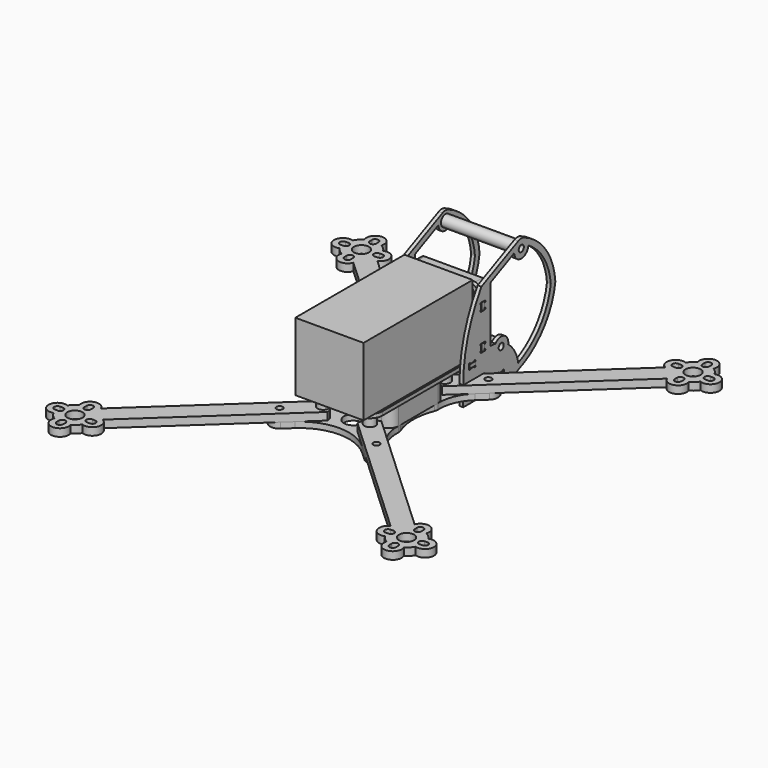
from build123d import *

# Parameters (mm, degrees)
F1_W      = 72
F1_H      = 36
F2_DEPTH  = 18
F4_R      = 1.7
F5_DEPTH  = 2
F7_R      = 1.7
F8_DEPTH  = 5
F13_R     = 1.7
F13_R_2   = 4
F14_DEPTH = 4
F16_R     = 1.7
F17_DEPTH = 10
F18_R     = 1.7
F18_R_2   = 5
F19_DEPTH = 3
F20_R     = 1.7
F21_DEPTH = 2
F24_R     = 1.7
F25_DEPTH = 2
F26_R     = 3
F26_R_2   = 1.7
F27_DEPTH = 6
F28_R     = 3
F28_R_2   = 1.7
F29_DEPTH = 38


# Not quite as in the source:
# - a feature names something its author has since deleted; it is built from what else it names


with BuildPart() as f2:
    # F1 (on Right) → F2 (new body, symmetric)
    with BuildSketch(Plane.YZ):
        with Locations((0, 23)):
            Rectangle(F1_W, F1_H)
    extrude(amount=F2_DEPTH, both=True)


with BuildPart() as f5:
    # F4 (on offset) → F5 (new body)
    with BuildSketch(Plane(origin=(0, 38, 0), x_dir=(-1, 0, 0), z_dir=(0, 1, 0))):
        with BuildLine():
            ThreePointArc((-15.25, 38), (-17.9016504294, 36.9016504294), (-19, 34.25))
            Line((-19, 34.25), (-19, 31.55))
            ThreePointArc((-19, 31.55), (-18.5, 31.05), (-19, 30.55))
            Line((-19, 30.55), (-21, 30.55))
            Line((-21, 30.55), (-21, 26.55))
            Line((-21, 26.55), (-19, 26.55))
            ThreePointArc((-19, 26.55), (-18.5, 26.05), (-19, 25.55))
            Line((-19, 25.55), (-19, 12.45))
            ThreePointArc((-19, 12.45), (-18.5, 11.95), (-19, 11.45))
            Line((-19, 11.45), (-21, 11.45))
            Line((-21, 11.45), (-21, 7.45))
            Line((-21, 7.45), (-19, 7.45))
            ThreePointArc((-19, 7.45), (-18.5, 6.95), (-19, 6.45))
            Line((-19, 6.45), (-19, 3.75))
            ThreePointArc((-19, 3.75), (-17.9016504294, 1.0983495706), (-15.25, 0))
            Line((-15.25, 0), (15.25, 0))
            ThreePointArc((15.25, 0), (17.9016504294, 1.0983495706), (19, 3.75))
            Line((19, 3.75), (19, 6.45))
            ThreePointArc((19, 6.45), (18.5, 6.95), (19, 7.45))
            Line((19, 7.45), (21, 7.45))
            Line((21, 7.45), (21, 11.45))
            Line((21, 11.45), (19, 11.45))
            ThreePointArc((19, 11.45), (18.5, 11.95), (19, 12.45))
            Line((19, 12.45), (19, 25.55))
            ThreePointArc((19, 25.55), (18.5, 26.05), (19, 26.55))
            Line((19, 26.55), (21, 26.55))
            Line((21, 26.55), (21, 30.55))
            Line((21, 30.55), (19, 30.55))
            ThreePointArc((19, 30.55), (18.5, 31.05), (19, 31.55))
            Line((19, 31.55), (19, 34.25))
            ThreePointArc((19, 34.25), (17.9016504294, 36.9016504294), (15.25, 38))
            Line((15.25, 38), (-15.25, 38))
        make_face()
        with Locations((-15.25, 3.75)):
            Circle(F4_R, mode=Mode.SUBTRACT)
        with Locations((15.25, 3.75)):
            Circle(F4_R, mode=Mode.SUBTRACT)
        with Locations((-15.25, 34.25)):
            Circle(F4_R, mode=Mode.SUBTRACT)
        with BuildLine():
            ThreePointArc((11.55, 34.25), (12.6337049096, 31.6337049096), (15.25, 30.55))
            Line((15.25, 30.55), (15.25, 7.45))
            ThreePointArc((15.25, 7.45), (12.6337049096, 6.3662950904), (11.55, 3.75))
            Line((11.55, 3.75), (-11.55, 3.75))
            ThreePointArc((-11.55, 3.75), (-12.6337049096, 6.3662950904), (-15.25, 7.45))
            Line((-15.25, 7.45), (-15.25, 30.55))
            ThreePointArc((-15.25, 30.55), (-12.6337049096, 31.6337049096), (-11.55, 34.25))
            Line((-11.55, 34.25), (11.55, 34.25))
        make_face(mode=Mode.SUBTRACT)
        with Locations((15.25, 34.25)):
            Circle(F4_R, mode=Mode.SUBTRACT)
    extrude(amount=F5_DEPTH)


with BuildPart() as f8:
    # F7 (on offset) → F8 (new body)
    with BuildSketch(Plane(origin=(0, 41, 0), x_dir=(-1, 0, 0), z_dir=(0, 1, 0))):
        with BuildLine():
            Line((15.25, 37), (-15.25, 37))
            ThreePointArc((-15.25, 37), (-17.1945436483, 36.1945436483), (-18, 34.25))
            Line((-18, 34.25), (-18, 3.75))
            ThreePointArc((-18, 3.75), (-17.1945436483, 1.8054563517), (-15.25, 1))
            Line((-15.25, 1), (15.25, 1))
            ThreePointArc((15.25, 1), (17.1945436483, 1.8054563517), (18, 3.75))
            Line((18, 3.75), (18, 34.25))
            ThreePointArc((18, 34.25), (17.1945436483, 36.1945436483), (15.25, 37))
        make_face()
        with Locations((-15.25, 3.75)):
            Circle(F7_R, mode=Mode.SUBTRACT)
        with Locations((15.25, 3.75)):
            Circle(F7_R, mode=Mode.SUBTRACT)
        with Locations((-15.25, 34.25)):
            Circle(F7_R, mode=Mode.SUBTRACT)
        with Locations((15.25, 34.25)):
            Circle(F7_R, mode=Mode.SUBTRACT)
    extrude(amount=F8_DEPTH)


with BuildPart() as f14:
    # F13 (on offset) → F14 (new body)
    with BuildSketch(Plane.XY.offset(-7)):
        with BuildLine():
            ThreePointArc((-13.5098647602, 23.45698286), (-13.5985378068, 25.8595100899), (-11.1960105769, 25.9481831366))
            Line((-11.1960105769, 25.9481831366), (-9.9504104386, 24.7912560449))
            ThreePointArc((-9.9504104386, 24.7912560449), (-8.9755957865, 24.5682394669), (-8.2950504384, 25.3009454306))
            Line((-8.2950504384, 25.3009454306), (-7.8315191856, 27.3270596371))
            Line((-7.8315191856, 27.3270596371), (-75.9697620511, 90.6146081253))
            ThreePointArc((-75.9697620511, 90.6146081253), (-77.7162022684, 90.1593612116), (-79.5054433115, 90.3958346237))
            ThreePointArc((-79.5054433115, 90.3958346237), (-80.9155407992, 88.3842819624), (-82.8176737402, 86.8297372354))
            ThreePointArc((-82.8176737402, 86.8297372354), (-82.4499479109, 85.0627961216), (-82.7752155315, 83.2875484882))
            Line((-82.7752155315, 83.2875484882), (-14.6369726661, 20))
            Line((-14.6369726661, 20), (-12.6505406659, 20.6116272629))
            ThreePointArc((-12.6505406659, 20.6116272629), (-11.9699953178, 21.3443332266), (-12.2642646219, 22.3000557683))
            Line((-12.2642646219, 22.3000557683), (-13.5098647602, 23.45698286))
        make_face()
        with Locations((-25.5416450153, 36.952399263)):
            Circle(F13_R, mode=Mode.SUBTRACT)
        with BuildLine():
            ThreePointArc((-79.5054433115, 90.3958346237), (-77.7162022684, 90.1593612116), (-75.9697620511, 90.6146081253))
            ThreePointArc((-75.9697620511, 90.6146081253), (-73.721275903, 96.7809760114), (-79.8297372354, 99.1823262598))
            ThreePointArc((-79.8297372354, 99.1823262598), (-81.3842819624, 101.0844592008), (-83.3958346237, 102.4945566885))
            ThreePointArc((-83.3958346237, 102.4945566885), (-88.0237403757, 108.6903381221), (-92.1823262598, 102.1702627646))
            ThreePointArc((-92.1823262598, 102.1702627646), (-94.0844592008, 100.6157180376), (-95.4945566885, 98.6041653763))
            ThreePointArc((-95.4945566885, 98.6041653763), (-101.6903381221, 93.9762596243), (-95.1702627646, 89.8176737402))
            ThreePointArc((-95.1702627646, 89.8176737402), (-93.6157180376, 87.9155407992), (-91.6041653763, 86.5054433115))
            ThreePointArc((-91.6041653763, 86.5054433115), (-88.7590568602, 80.5906195275), (-82.7752155315, 83.2875484882))
            ThreePointArc((-82.7752155315, 83.2875484882), (-82.4499479109, 85.0627961216), (-82.8176737402, 86.8297372354))
            ThreePointArc((-82.8176737402, 86.8297372354), (-80.9155407992, 88.3842819624), (-79.5054433115, 90.3958346237))
        make_face()
        with BuildLine():
            ThreePointArc((-96.930834755, 92.4507670157), (-98.6923793639, 94.0869089994), (-97.0562373802, 95.8484536083))
            Line((-97.0562373802, 95.8484536083), (-95.5572580011, 95.9037782959))
            ThreePointArc((-95.5572580011, 95.9037782959), (-93.7957133922, 94.2676363122), (-95.4318553759, 92.5060917033))
            Line((-95.4318553759, 92.5060917033), (-96.930834755, 92.4507670157))
        make_face(mode=Mode.SUBTRACT)
        with BuildLine():
            ThreePointArc((-85.4507670157, 85.069165245), (-87.0869089994, 83.3076206361), (-88.8484536083, 84.9437626198))
            Line((-88.8484536083, 84.9437626198), (-88.9037782959, 86.4427419989))
            ThreePointArc((-88.9037782959, 86.4427419989), (-87.2676363122, 88.2042866078), (-85.5060917033, 86.5681446241))
            Line((-85.5060917033, 86.5681446241), (-85.4507670157, 85.069165245))
        make_face(mode=Mode.SUBTRACT)
        with Locations((-87.5, 94.5)):
            Circle(F13_R_2, mode=Mode.SUBTRACT)
        with BuildLine():
            ThreePointArc((-78.069165245, 96.5492329843), (-76.3076206361, 94.9130910006), (-77.9437626198, 93.1515463917))
            Line((-77.9437626198, 93.1515463917), (-79.4427419989, 93.0962217041))
            ThreePointArc((-79.4427419989, 93.0962217041), (-81.2042866078, 94.7323636878), (-79.5681446241, 96.4939082967))
            Line((-79.5681446241, 96.4939082967), (-78.069165245, 96.5492329843))
        make_face(mode=Mode.SUBTRACT)
        with BuildLine():
            Line((-89.4939082967, 102.4318553759), (-89.5492329843, 103.930834755))
            ThreePointArc((-89.5492329843, 103.930834755), (-87.9130910006, 105.6923793639), (-86.1515463917, 104.0562373802))
            Line((-86.1515463917, 104.0562373802), (-86.0962217041, 102.5572580011))
            ThreePointArc((-86.0962217041, 102.5572580011), (-87.7323636878, 100.7957133922), (-89.4939082967, 102.4318553759))
        make_face(mode=Mode.SUBTRACT)
    extrude(amount=F14_DEPTH)


with BuildPart() as f14b:
    # F13 (on offset) → F14, piece 2 (new body)
    with BuildSketch(Plane.XY.offset(-7)):
        with BuildLine():
            Line((75.9697620511, 90.6146081253), (7.8315191856, 27.3270596371))
            Line((7.8315191856, 27.3270596371), (8.2950504384, 25.3009454306))
            ThreePointArc((8.2950504384, 25.3009454306), (8.9755957865, 24.5682394669), (9.9504104386, 24.7912560449))
            Line((9.9504104386, 24.7912560449), (11.1960105769, 25.9481831366))
            ThreePointArc((11.1960105769, 25.9481831366), (13.5985378068, 25.8595100899), (13.5098647602, 23.45698286))
            Line((13.5098647602, 23.45698286), (12.2642646219, 22.3000557683))
            ThreePointArc((12.2642646219, 22.3000557683), (11.9699953178, 21.3443332266), (12.6505406659, 20.6116272629))
            Line((12.6505406659, 20.6116272629), (14.6369726661, 20))
            Line((14.6369726661, 20), (82.7752155315, 83.2875484882))
            ThreePointArc((82.7752155315, 83.2875484882), (82.4499479109, 85.0627961216), (82.8176737402, 86.8297372354))
            ThreePointArc((82.8176737402, 86.8297372354), (80.9155407992, 88.3842819624), (79.5054433115, 90.3958346237))
            ThreePointArc((79.5054433115, 90.3958346237), (77.7162022684, 90.1593612116), (75.9697620511, 90.6146081253))
        make_face()
        with Locations((25.5416450153, 36.952399263)):
            Circle(F13_R, mode=Mode.SUBTRACT)
        with BuildLine():
            ThreePointArc((79.8297372354, 99.1823262598), (73.721275903, 96.7809760114), (75.9697620511, 90.6146081253))
            ThreePointArc((75.9697620511, 90.6146081253), (77.7162022684, 90.1593612116), (79.5054433115, 90.3958346237))
            ThreePointArc((79.5054433115, 90.3958346237), (80.9155407992, 88.3842819624), (82.8176737402, 86.8297372354))
            ThreePointArc((82.8176737402, 86.8297372354), (82.4499479109, 85.0627961216), (82.7752155315, 83.2875484882))
            ThreePointArc((82.7752155315, 83.2875484882), (88.7590568602, 80.5906195275), (91.6041653763, 86.5054433115))
            ThreePointArc((91.6041653763, 86.5054433115), (93.6157180376, 87.9155407992), (95.1702627646, 89.8176737402))
            ThreePointArc((95.1702627646, 89.8176737402), (101.6903381221, 93.9762596243), (95.4945566885, 98.6041653763))
            ThreePointArc((95.4945566885, 98.6041653763), (94.0844592008, 100.6157180376), (92.1823262598, 102.1702627646))
            ThreePointArc((92.1823262598, 102.1702627646), (88.0237403757, 108.6903381221), (83.3958346237, 102.4945566885))
            ThreePointArc((83.3958346237, 102.4945566885), (81.3842819624, 101.0844592008), (79.8297372354, 99.1823262598))
        make_face()
        with BuildLine():
            Line((88.9037782959, 86.4427419989), (88.8484536083, 84.9437626198))
            ThreePointArc((88.8484536083, 84.9437626198), (87.0869089994, 83.3076206361), (85.4507670157, 85.069165245))
            Line((85.4507670157, 85.069165245), (85.5060917033, 86.5681446241))
            ThreePointArc((85.5060917033, 86.5681446241), (87.2676363122, 88.2042866078), (88.9037782959, 86.4427419989))
        make_face(mode=Mode.SUBTRACT)
        with BuildLine():
            Line((78.069165245, 96.5492329843), (79.5681446241, 96.4939082967))
            ThreePointArc((79.5681446241, 96.4939082967), (81.2042866078, 94.7323636878), (79.4427419989, 93.0962217041))
            Line((79.4427419989, 93.0962217041), (77.9437626198, 93.1515463917))
            ThreePointArc((77.9437626198, 93.1515463917), (76.3076206361, 94.9130910006), (78.069165245, 96.5492329843))
        make_face(mode=Mode.SUBTRACT)
        with Locations((87.5, 94.5)):
            Circle(F13_R_2, mode=Mode.SUBTRACT)
        with BuildLine():
            Line((95.5572580011, 95.9037782959), (97.0562373802, 95.8484536083))
            ThreePointArc((97.0562373802, 95.8484536083), (98.6923793639, 94.0869089994), (96.930834755, 92.4507670157))
            Line((96.930834755, 92.4507670157), (95.4318553759, 92.5060917033))
            ThreePointArc((95.4318553759, 92.5060917033), (93.7957133922, 94.2676363122), (95.5572580011, 95.9037782959))
        make_face(mode=Mode.SUBTRACT)
        with BuildLine():
            Line((86.0962217041, 102.5572580011), (86.1515463917, 104.0562373802))
            ThreePointArc((86.1515463917, 104.0562373802), (87.9130910006, 105.6923793639), (89.5492329843, 103.930834755))
            Line((89.5492329843, 103.930834755), (89.4939082967, 102.4318553759))
            ThreePointArc((89.4939082967, 102.4318553759), (87.7323636878, 100.7957133922), (86.0962217041, 102.5572580011))
        make_face(mode=Mode.SUBTRACT)
    extrude(amount=F14_DEPTH)


with BuildPart() as f14c:
    # F13 (on offset) → F14, piece 3 (new body)
    with BuildSketch(Plane.XY.offset(-7)):
        with BuildLine():
            ThreePointArc((13.5098647602, -23.45698286), (13.5985378068, -25.8595100899), (11.1960105769, -25.9481831366))
            Line((11.1960105769, -25.9481831366), (9.9504104386, -24.7912560449))
            ThreePointArc((9.9504104386, -24.7912560449), (8.9755957865, -24.5682394669), (8.2950504384, -25.3009454306))
            Line((8.2950504384, -25.3009454306), (7.8315191856, -27.3270596371))
            Line((7.8315191856, -27.3270596371), (75.9697620511, -90.6146081253))
            ThreePointArc((75.9697620511, -90.6146081253), (77.7162022684, -90.1593612116), (79.5054433115, -90.3958346237))
            ThreePointArc((79.5054433115, -90.3958346237), (80.9155407992, -88.3842819624), (82.8176737402, -86.8297372354))
            ThreePointArc((82.8176737402, -86.8297372354), (82.4499479109, -85.0627961216), (82.7752155315, -83.2875484882))
            Line((82.7752155315, -83.2875484882), (14.6369726661, -20))
            Line((14.6369726661, -20), (12.6505406659, -20.6116272629))
            ThreePointArc((12.6505406659, -20.6116272629), (11.9699953178, -21.3443332266), (12.2642646219, -22.3000557683))
            Line((12.2642646219, -22.3000557683), (13.5098647602, -23.45698286))
        make_face()
        with Locations((25.5416450153, -36.952399263)):
            Circle(F13_R, mode=Mode.SUBTRACT)
        with BuildLine():
            ThreePointArc((79.5054433115, -90.3958346237), (77.7162022684, -90.1593612116), (75.9697620511, -90.6146081253))
            ThreePointArc((75.9697620511, -90.6146081253), (73.721275903, -96.7809760114), (79.8297372354, -99.1823262598))
            ThreePointArc((79.8297372354, -99.1823262598), (81.3842819624, -101.0844592008), (83.3958346237, -102.4945566885))
            ThreePointArc((83.3958346237, -102.4945566885), (88.0237403757, -108.6903381221), (92.1823262598, -102.1702627646))
            ThreePointArc((92.1823262598, -102.1702627646), (94.0844592008, -100.6157180376), (95.4945566885, -98.6041653763))
            ThreePointArc((95.4945566885, -98.6041653763), (101.6903381221, -93.9762596243), (95.1702627646, -89.8176737402))
            ThreePointArc((95.1702627646, -89.8176737402), (93.6157180376, -87.9155407992), (91.6041653763, -86.5054433115))
            ThreePointArc((91.6041653763, -86.5054433115), (88.7590568602, -80.5906195275), (82.7752155315, -83.2875484882))
            ThreePointArc((82.7752155315, -83.2875484882), (82.4499479109, -85.0627961216), (82.8176737402, -86.8297372354))
            ThreePointArc((82.8176737402, -86.8297372354), (80.9155407992, -88.3842819624), (79.5054433115, -90.3958346237))
        make_face()
        with BuildLine():
            Line((89.4939082967, -102.4318553759), (89.5492329843, -103.930834755))
            ThreePointArc((89.5492329843, -103.930834755), (87.9130910006, -105.6923793639), (86.1515463917, -104.0562373802))
            Line((86.1515463917, -104.0562373802), (86.0962217041, -102.5572580011))
            ThreePointArc((86.0962217041, -102.5572580011), (87.7323636878, -100.7957133922), (89.4939082967, -102.4318553759))
        make_face(mode=Mode.SUBTRACT)
        with BuildLine():
            ThreePointArc((79.4427419989, -93.0962217041), (81.2042866078, -94.7323636878), (79.5681446241, -96.4939082967))
            Line((79.5681446241, -96.4939082967), (78.069165245, -96.5492329843))
            ThreePointArc((78.069165245, -96.5492329843), (76.3076206361, -94.9130910006), (77.9437626198, -93.1515463917))
            Line((77.9437626198, -93.1515463917), (79.4427419989, -93.0962217041))
        make_face(mode=Mode.SUBTRACT)
        with Locations((87.5, -94.5)):
            Circle(F13_R_2, mode=Mode.SUBTRACT)
        with BuildLine():
            Line((88.8484536083, -84.9437626198), (88.9037782959, -86.4427419989))
            ThreePointArc((88.9037782959, -86.4427419989), (87.2676363122, -88.2042866078), (85.5060917033, -86.5681446241))
            Line((85.5060917033, -86.5681446241), (85.4507670157, -85.069165245))
            ThreePointArc((85.4507670157, -85.069165245), (87.0869089994, -83.3076206361), (88.8484536083, -84.9437626198))
        make_face(mode=Mode.SUBTRACT)
        with BuildLine():
            ThreePointArc((95.5572580011, -95.9037782959), (93.7957133922, -94.2676363122), (95.4318553759, -92.5060917033))
            Line((95.4318553759, -92.5060917033), (96.930834755, -92.4507670157))
            ThreePointArc((96.930834755, -92.4507670157), (98.6923793639, -94.0869089994), (97.0562373802, -95.8484536083))
            Line((97.0562373802, -95.8484536083), (95.5572580011, -95.9037782959))
        make_face(mode=Mode.SUBTRACT)
    extrude(amount=F14_DEPTH)


with BuildPart() as f14d:
    # F13 (on offset) → F14, piece 4 (new body)
    with BuildSketch(Plane.XY.offset(-7)):
        with BuildLine():
            Line((-9.9504104386, -24.7912560449), (-11.1960105769, -25.9481831366))
            ThreePointArc((-11.1960105769, -25.9481831366), (-13.5985378068, -25.8595100899), (-13.5098647602, -23.45698286))
            Line((-13.5098647602, -23.45698286), (-12.2642646219, -22.3000557683))
            ThreePointArc((-12.2642646219, -22.3000557683), (-11.9699953178, -21.3443332266), (-12.6505406659, -20.6116272629))
            Line((-12.6505406659, -20.6116272629), (-14.6369726661, -20))
            Line((-14.6369726661, -20), (-82.7752155315, -83.2875484882))
            ThreePointArc((-82.7752155315, -83.2875484882), (-82.4499479109, -85.0627961216), (-82.8176737402, -86.8297372354))
            ThreePointArc((-82.8176737402, -86.8297372354), (-80.9155407992, -88.3842819624), (-79.5054433115, -90.3958346237))
            ThreePointArc((-79.5054433115, -90.3958346237), (-77.7162022684, -90.1593612116), (-75.9697620511, -90.6146081253))
            Line((-75.9697620511, -90.6146081253), (-7.8315191856, -27.3270596371))
            Line((-7.8315191856, -27.3270596371), (-8.2950504384, -25.3009454306))
            ThreePointArc((-8.2950504384, -25.3009454306), (-8.9755957865, -24.5682394669), (-9.9504104386, -24.7912560449))
        make_face()
        with Locations((-25.5416450153, -36.952399263)):
            Circle(F13_R, mode=Mode.SUBTRACT)
        with BuildLine():
            ThreePointArc((-79.8297372354, -99.1823262598), (-73.721275903, -96.7809760114), (-75.9697620511, -90.6146081253))
            ThreePointArc((-75.9697620511, -90.6146081253), (-77.7162022684, -90.1593612116), (-79.5054433115, -90.3958346237))
            ThreePointArc((-79.5054433115, -90.3958346237), (-80.9155407992, -88.3842819624), (-82.8176737402, -86.8297372354))
            ThreePointArc((-82.8176737402, -86.8297372354), (-82.4499479109, -85.0627961216), (-82.7752155315, -83.2875484882))
            ThreePointArc((-82.7752155315, -83.2875484882), (-88.7590568602, -80.5906195275), (-91.6041653763, -86.5054433115))
            ThreePointArc((-91.6041653763, -86.5054433115), (-93.6157180376, -87.9155407992), (-95.1702627646, -89.8176737402))
            ThreePointArc((-95.1702627646, -89.8176737402), (-101.6903381221, -93.9762596243), (-95.4945566885, -98.6041653763))
            ThreePointArc((-95.4945566885, -98.6041653763), (-94.0844592008, -100.6157180376), (-92.1823262598, -102.1702627646))
            ThreePointArc((-92.1823262598, -102.1702627646), (-88.0237403757, -108.6903381221), (-83.3958346237, -102.4945566885))
            ThreePointArc((-83.3958346237, -102.4945566885), (-81.3842819624, -101.0844592008), (-79.8297372354, -99.1823262598))
        make_face()
        with BuildLine():
            Line((-86.0962217041, -102.5572580011), (-86.1515463917, -104.0562373802))
            ThreePointArc((-86.1515463917, -104.0562373802), (-87.9130910006, -105.6923793639), (-89.5492329843, -103.930834755))
            Line((-89.5492329843, -103.930834755), (-89.4939082967, -102.4318553759))
            ThreePointArc((-89.4939082967, -102.4318553759), (-87.7323636878, -100.7957133922), (-86.0962217041, -102.5572580011))
        make_face(mode=Mode.SUBTRACT)
        with BuildLine():
            Line((-96.930834755, -92.4507670157), (-95.4318553759, -92.5060917033))
            ThreePointArc((-95.4318553759, -92.5060917033), (-93.7957133922, -94.2676363122), (-95.5572580011, -95.9037782959))
            Line((-95.5572580011, -95.9037782959), (-97.0562373802, -95.8484536083))
            ThreePointArc((-97.0562373802, -95.8484536083), (-98.6923793639, -94.0869089994), (-96.930834755, -92.4507670157))
        make_face(mode=Mode.SUBTRACT)
        with Locations((-87.5, -94.5)):
            Circle(F13_R_2, mode=Mode.SUBTRACT)
        with BuildLine():
            Line((-79.4427419989, -93.0962217041), (-77.9437626198, -93.1515463917))
            ThreePointArc((-77.9437626198, -93.1515463917), (-76.3076206361, -94.9130910006), (-78.069165245, -96.5492329843))
            Line((-78.069165245, -96.5492329843), (-79.5681446241, -96.4939082967))
            ThreePointArc((-79.5681446241, -96.4939082967), (-81.2042866078, -94.7323636878), (-79.4427419989, -93.0962217041))
        make_face(mode=Mode.SUBTRACT)
        with BuildLine():
            ThreePointArc((-85.5060917033, -86.5681446241), (-87.2676363122, -88.2042866078), (-88.9037782959, -86.4427419989))
            Line((-88.9037782959, -86.4427419989), (-88.8484536083, -84.9437626198))
            ThreePointArc((-88.8484536083, -84.9437626198), (-87.0869089994, -83.3076206361), (-85.4507670157, -85.069165245))
            Line((-85.4507670157, -85.069165245), (-85.5060917033, -86.5681446241))
        make_face(mode=Mode.SUBTRACT)
    extrude(amount=F14_DEPTH)


with BuildPart() as f17:
    # F16 (on offset) → F17 (new body)
    with BuildSketch(Plane.XY.offset(-7)):
        with BuildLine():
            Line((13, 18), (-13, 18))
            ThreePointArc((-13, 18), (-16.5355339059, 16.5355339059), (-18, 13))
            Line((-18, 13), (-18, -13))
            ThreePointArc((-18, -13), (-16.5355339059, -16.5355339059), (-13, -18))
            Line((-13, -18), (13, -18))
            ThreePointArc((13, -18), (16.5355339059, -16.5355339059), (18, -13))
            Line((18, -13), (18, 13))
            ThreePointArc((18, 13), (16.5355339059, 16.5355339059), (13, 18))
        make_face()
        with Locations((-13, -13)):
            Circle(F16_R, mode=Mode.SUBTRACT)
        with Locations((13, -13)):
            Circle(F16_R, mode=Mode.SUBTRACT)
        with Locations((-13, 13)):
            Circle(F16_R, mode=Mode.SUBTRACT)
        with Locations((13, 13)):
            Circle(F16_R, mode=Mode.SUBTRACT)
    extrude(amount=F17_DEPTH)


with BuildPart() as f19:
    # F18 (on offset) → F19 (new body)
    with BuildSketch(Plane.XY.offset(-7)):
        with BuildLine():
            ThreePointArc((-22.1389175981, 40.6159284527), (-29.2051745195, 40.3551263418), (-28.9443717555, 33.2888694445))
            Line((-28.9443717555, 33.2888694445), (-24.5481359733, 29.2055973562))
            ThreePointArc((-24.5481359733, 29.2055973562), (-19.4694285614, 21.8319926769), (-18, 13))
            ThreePointArc((-18, 13), (-17.9097626368, 12.0543621991), (-17.6423076598, 11.1428571429))
            ThreePointArc((-17.6423076598, 11.1428571429), (-15.4961536185, 0), (-17.6423076598, -11.1428571429))
            ThreePointArc((-17.6423076598, -11.1428571429), (-17.9097627454, -12.0543627633), (-18, -13.0000011492))
            ThreePointArc((-18, -13.0000011492), (-19.4694287941, -21.8319932092), (-24.5481359733, -29.2055973562))
            Line((-24.5481359733, -29.2055973562), (-28.9443717555, -33.2888694445))
            ThreePointArc((-28.9443717555, -33.2888694445), (-29.2051745195, -40.3551263418), (-22.1389175981, -40.6159284527))
            Line((-22.1389175981, -40.6159284527), (-17.7426825704, -36.532655552))
            ThreePointArc((-17.7426825704, -36.532655552), (0, -29.563958256), (17.7426825704, -36.532655552))
            Line((17.7426825704, -36.532655552), (22.1389175981, -40.6159284527))
            ThreePointArc((22.1389175981, -40.6159284527), (29.2051745195, -40.3551263418), (28.9443717555, -33.2888694445))
            Line((28.9443717555, -33.2888694445), (24.5481359733, -29.2055973562))
            ThreePointArc((24.5481359733, -29.2055973562), (19.4694287941, -21.8319932092), (18, -13.0000011492))
            ThreePointArc((18, -13.0000011492), (17.9097627454, -12.0543627633), (17.6423076598, -11.1428571429))
            ThreePointArc((17.6423076598, -11.1428571429), (15.4961536185, 0), (17.6423076598, 11.1428571429))
            ThreePointArc((17.6423076598, 11.1428571429), (17.9097626368, 12.0543621991), (18, 13))
            ThreePointArc((18, 13), (19.4694285614, 21.8319926769), (24.5481359733, 29.2055973562))
            Line((24.5481359733, 29.2055973562), (28.9443717555, 33.2888694445))
            ThreePointArc((28.9443717555, 33.2888694445), (29.2051745195, 40.3551263418), (22.1389175981, 40.6159284527))
            Line((22.1389175981, 40.6159284527), (19, 37.7004662254))
            Line((19, 37.7004662254), (19, 47.7004662254))
            ThreePointArc((19, 47.7004662254), (18.5, 48.2004662254), (19, 48.7004662254))
            Line((19, 48.7004662254), (21, 48.7004662254))
            Line((21, 48.7004662254), (21, 52.7004662254))
            Line((21, 52.7004662254), (19, 52.7004662254))
            ThreePointArc((19, 52.7004662254), (18.5, 53.2004662254), (19, 53.7004662254))
            Line((19, 53.7004662254), (19, 56.7004662254))
            ThreePointArc((19, 56.7004662254), (17.4351844247, 58.6525457618), (15.1893854835, 57.5499808353))
            Line((15.1893854835, 57.5499808353), (4.5265362913, 34.823697722))
            ThreePointArc((4.5265362913, 34.823697722), (0, 31.9474842469), (-4.5265362913, 34.823697722))
            Line((-4.5265362913, 34.823697722), (-15.1893854835, 57.5499808353))
            ThreePointArc((-15.1893854835, 57.5499808353), (-17.4351844247, 58.6525457618), (-19, 56.7004662254))
            Line((-19, 56.7004662254), (-19, 53.7004662254))
            ThreePointArc((-19, 53.7004662254), (-18.5, 53.2004662254), (-19, 52.7004662254))
            Line((-19, 52.7004662254), (-21, 52.7004662254))
            Line((-21, 52.7004662254), (-21, 48.7004662254))
            Line((-21, 48.7004662254), (-19, 48.7004662254))
            ThreePointArc((-19, 48.7004662254), (-18.5, 48.2004662254), (-19, 47.7004662254))
            Line((-19, 47.7004662254), (-19, 37.7004662254))
            Line((-19, 37.7004662254), (-22.1389175981, 40.6159284527))
        make_face()
        with Locations((-25.5416450153, -36.952399263)):
            Circle(F18_R, mode=Mode.SUBTRACT)
        with Locations((-13, -13)):
            Circle(F18_R, mode=Mode.SUBTRACT)
        with Locations((0, -20.1760563247)):
            Circle(F18_R_2, mode=Mode.SUBTRACT)
        with Locations((25.5416450153, -36.952399263)):
            Circle(F18_R, mode=Mode.SUBTRACT)
        with Locations((13, -13)):
            Circle(F18_R, mode=Mode.SUBTRACT)
        Circle(F18_R_2, mode=Mode.SUBTRACT)
        with Locations((-13, 13)):
            Circle(F18_R, mode=Mode.SUBTRACT)
        with Locations((-25.5416450153, 36.952399263)):
            Circle(F18_R, mode=Mode.SUBTRACT)
        with Locations((0, 20.1760563247)):
            Circle(F18_R_2, mode=Mode.SUBTRACT)
        with Locations((13, 13)):
            Circle(F18_R, mode=Mode.SUBTRACT)
        with Locations((25.5416450153, 36.952399263)):
            Circle(F18_R, mode=Mode.SUBTRACT)
    extrude(amount=-F19_DEPTH)


with BuildPart() as f21:
    # F20 (on offset) → F21 (new body)
    with BuildSketch(Plane.YZ.offset(-19)):
        with BuildLine():
            Line((62.3282767321, 49.3444617499), (38, 38))
            ThreePointArc((38, 38), (29.0826290872, 18.4320000233), (26, -2.85))
            Line((26, -2.85), (40, -2.85))
            Line((40, -2.85), (40, -10.15))
            Line((40, -10.15), (26, -10.15))
            Line((26, -10.15), (26, -13.15))
            Line((26, -13.15), (40, -13.15))
            Line((40, -13.15), (48.152460205, -13.15))
            ThreePointArc((48.152460205, -13.15), (73.7471319214, -3.5814468486), (86.7876259061, 20.4308405543))
            ThreePointArc((86.7876259061, 20.4308405543), (80.5806098218, 37.8584878255), (66.1362156447, 49.4174417114))
            ThreePointArc((66.1362156447, 49.4174417114), (68.2294053863, 47.6856154616), (69.0145825623, 45.0848151508))
            ThreePointArc((69.0145825623, 45.0848151508), (69.0084593346, 44.8449801113), (68.9901056065, 44.6057699929))
            ThreePointArc((68.9901056065, 44.6057699929), (79.2518042963, 34.4400457254), (83.7587593166, 20.7166435843))
            ThreePointArc((83.7587593166, 20.7166435843), (76.6748400327, 3.938531383), (62.2816739433, -7.2204887973))
            ThreePointArc((62.2816739433, -7.2204887973), (60.0266628863, -0.9746693905), (55.6739003109, 4.0401878249))
            ThreePointArc((55.6739003109, 4.0401878249), (49.1433099786, 0.5733712966), (47.3258138651, 7.7402489157))
            ThreePointArc((47.3258138651, 7.7402489157), (45.7431345689, 7.928925637), (44.15, 7.9778634036))
            Line((44.15, 7.9778634036), (44.15, 37.5576583408))
            Line((44.15, 37.5576583408), (59.6248897653, 44.7737179474))
            ThreePointArc((59.6248897653, 44.7737179474), (60.2691945532, 47.4774780723), (62.3282767321, 49.3444617499))
        make_face()
        with BuildLine():
            ThreePointArc((51.8504662254, -6.85), (52.3504662254, -6.35), (52.8504662254, -6.85))
            Line((52.8504662254, -6.85), (52.8504662254, -10.15))
            ThreePointArc((52.8504662254, -10.15), (52.3504662254, -10.65), (51.8504662254, -10.15))
            Line((51.8504662254, -10.15), (49.5504662254, -10.15))
            ThreePointArc((49.5504662254, -10.15), (49.0504662254, -10.65), (48.5504662254, -10.15))
            Line((48.5504662254, -10.15), (48.5504662254, -6.85))
            ThreePointArc((48.5504662254, -6.85), (49.0504662254, -6.35), (49.5504662254, -6.85))
            Line((49.5504662254, -6.85), (51.8504662254, -6.85))
        make_face(mode=Mode.SUBTRACT)
        with BuildLine():
            ThreePointArc((33.15, 5.15), (33.65, 5.65), (34.15, 5.15))
            Line((34.15, 5.15), (34.15, 2.85))
            ThreePointArc((34.15, 2.85), (33.65, 2.35), (33.15, 2.85))
            Line((33.15, 2.85), (30.85, 2.85))
            ThreePointArc((30.85, 2.85), (30.35, 2.35), (29.85, 2.85))
            Line((29.85, 2.85), (29.85, 5.15))
            ThreePointArc((29.85, 5.15), (30.35, 5.65), (30.85, 5.15))
            Line((30.85, 5.15), (33.15, 5.15))
        make_face(mode=Mode.SUBTRACT)
        with BuildLine():
            Line((37.85, 11.6), (40.15, 11.6))
            ThreePointArc((40.15, 11.6), (40.65, 11.1), (40.15, 10.6))
            Line((40.15, 10.6), (40.15, 8.3))
            ThreePointArc((40.15, 8.3), (40.65, 7.8), (40.15, 7.3))
            Line((40.15, 7.3), (37.85, 7.3))
            ThreePointArc((37.85, 7.3), (37.35, 7.8), (37.85, 8.3))
            Line((37.85, 8.3), (37.85, 10.6))
            ThreePointArc((37.85, 10.6), (37.35, 11.1), (37.85, 11.6))
        make_face(mode=Mode.SUBTRACT)
        with BuildLine():
            Line((37.85, 30.7), (40.15, 30.7))
            ThreePointArc((40.15, 30.7), (40.65, 30.2), (40.15, 29.7))
            Line((40.15, 29.7), (40.15, 27.4))
            ThreePointArc((40.15, 27.4), (40.65, 26.9), (40.15, 26.4))
            Line((40.15, 26.4), (37.85, 26.4))
            ThreePointArc((37.85, 26.4), (37.35, 26.9), (37.85, 27.4))
            Line((37.85, 27.4), (37.85, 29.7))
            ThreePointArc((37.85, 29.7), (37.35, 30.2), (37.85, 30.7))
        make_face(mode=Mode.SUBTRACT)
        with BuildLine():
            ThreePointArc((55.7477758944, 4.870231729), (52.5638198354, 9.3190080517), (47.3258138651, 7.7402489157))
            ThreePointArc((47.3258138651, 7.7402489157), (49.1433099786, 0.5733712966), (55.6739003109, 4.0401878249))
            ThreePointArc((55.6739003109, 4.0401878249), (55.729270568, 4.4535692503), (55.7477758944, 4.870231729))
        make_face()
        with Locations((51.0477758944, 4.870231729)):
            Circle(F20_R, mode=Mode.SUBTRACT)
        with BuildLine():
            ThreePointArc((66.1362156447, 49.4174417114), (64.2245225981, 49.7839522208), (62.3282767321, 49.3444617499))
            ThreePointArc((62.3282767321, 49.3444617499), (60.2691945532, 47.4774780723), (59.6248897653, 44.7737179474))
            ThreePointArc((59.6248897653, 44.7737179474), (64.2303102399, 40.3855707248), (68.9901056065, 44.6057699929))
            ThreePointArc((68.9901056065, 44.6057699929), (69.0084593346, 44.8449801113), (69.0145825623, 45.0848151508))
            ThreePointArc((69.0145825623, 45.0848151508), (68.2294053863, 47.6856154616), (66.1362156447, 49.4174417114))
        make_face()
        with Locations((64.3145825623, 45.0848151508)):
            Circle(F20_R, mode=Mode.SUBTRACT)
    extrude(amount=-F21_DEPTH)


with BuildPart() as f22_1:
    # F22: instance of F21
    add(f21.part.mirror(Plane.YZ))


with BuildPart() as f25:
    # F24 (on offset) → F25 (new body)
    with BuildSketch(Plane.XY.offset(3)):
        with BuildLine():
            ThreePointArc((-19, -24.7025829983), (-17.0531205181, -29.4027658478), (-12.3529376685, -31.3496453297))
            Line((-12.3529376685, -31.3496453297), (12.3529376685, -31.3496453297))
            ThreePointArc((12.3529376685, -31.3496453297), (17.0531205181, -29.4027658478), (19, -24.7025829983))
            Line((19, -24.7025829983), (19, 29))
            ThreePointArc((19, 29), (18.5, 29.5), (19, 30))
            Line((19, 30), (21, 30))
            Line((21, 30), (21, 34))
            Line((21, 34), (-21, 34))
            Line((-21, 34), (-21, 30))
            Line((-21, 30), (-19, 30))
            ThreePointArc((-19, 30), (-18.5, 29.5), (-19, 29))
            Line((-19, 29), (-19, -24.7025829983))
        make_face()
        with Locations((-12.3529376685, -24.7025829983)):
            Circle(F24_R, mode=Mode.SUBTRACT)
        Polygon((-15, -10), (-15, 10), (-2.4115464281, 0), align=None, mode=Mode.SUBTRACT)
        with Locations((12.3529376685, -24.7025829983)):
            Circle(F24_R, mode=Mode.SUBTRACT)
        with BuildLine():
            ThreePointArc((-7.3048626876, -27.3496453297), (-8.3224290158, -20.6720743455), (-15, -19.6545080173))
            Line((-15, -19.6545080173), (-15, -13.8313624693))
            Line((-15, -13.8313624693), (0, -1.9156812347))
            Line((0, -1.9156812347), (15, -13.8313624693))
            Line((15, -13.8313624693), (15, -19.6545080173))
            ThreePointArc((15, -19.6545080173), (8.3224290158, -20.6720743455), (7.3048626876, -27.3496453297))
            Line((7.3048626876, -27.3496453297), (-7.3048626876, -27.3496453297))
        make_face(mode=Mode.SUBTRACT)
        Polygon((2.4115464281, 0), (15, 10), (15, -10), align=None, mode=Mode.SUBTRACT)
        with Locations((-12.3529376685, 24.7025829983)):
            Circle(F24_R, mode=Mode.SUBTRACT)
        with BuildLine():
            ThreePointArc((-15, 19.6545080173), (-7.1730733535, 22.323716529), (-10.2488052797, 30))
            Line((-10.2488052797, 30), (10.2488052797, 30))
            ThreePointArc((10.2488052797, 30), (7.1730733535, 22.323716529), (15, 19.6545080173))
            Line((15, 19.6545080173), (15, 13.8313624693))
            Line((15, 13.8313624693), (0, 1.9156812347))
            Line((0, 1.9156812347), (-15, 13.8313624693))
            Line((-15, 13.8313624693), (-15, 19.6545080173))
        make_face(mode=Mode.SUBTRACT)
        with Locations((12.3529376685, 24.7025829983)):
            Circle(F24_R, mode=Mode.SUBTRACT)
    extrude(amount=F25_DEPTH)


with BuildPart() as f27:
    # F26 (on offset) → F27 (new body)
    with BuildSketch(Plane.XY.offset(-3)):
        with Locations((-12.3529376685, 24.7025829983)):
            Circle(F26_R)
        with Locations((-12.3529376685, 24.7025829983)):
            Circle(F26_R_2, mode=Mode.SUBTRACT)
    extrude(amount=F27_DEPTH)


with BuildPart() as f27b:
    # F26 (on offset) → F27, piece 2 (new body)
    with BuildSketch(Plane.XY.offset(-3)):
        with Locations((12.3529376685, 24.7025829983)):
            Circle(F26_R)
        with Locations((12.3529376685, 24.7025829983)):
            Circle(F26_R_2, mode=Mode.SUBTRACT)
    extrude(amount=F27_DEPTH)


with BuildPart() as f27c:
    # F26 (on offset) → F27, piece 3 (new body)
    with BuildSketch(Plane.XY.offset(-3)):
        with Locations((12.3529376685, -24.7025829983)):
            Circle(F26_R)
        with Locations((12.3529376685, -24.7025829983)):
            Circle(F26_R_2, mode=Mode.SUBTRACT)
    extrude(amount=F27_DEPTH)


with BuildPart() as f27d:
    # F26 (on offset) → F27, piece 4 (new body)
    with BuildSketch(Plane.XY.offset(-3)):
        with Locations((-12.3529376685, -24.7025829983)):
            Circle(F26_R)
        with Locations((-12.3529376685, -24.7025829983)):
            Circle(F26_R_2, mode=Mode.SUBTRACT)
    extrude(amount=F27_DEPTH)


with BuildPart() as f29:
    # F28 (on face) → F29 (new body)
    with BuildSketch(Plane.YZ.offset(-19)):
        with Locations((51.0477758944, 4.870231729)):
            Circle(F28_R)
        with Locations((51.0477758944, 4.870231729)):
            Circle(F28_R_2, mode=Mode.SUBTRACT)
    extrude(amount=F29_DEPTH)


with BuildPart() as f29b:
    # F28 (on face) → F29, piece 2 (new body)
    with BuildSketch(Plane.YZ.offset(-19)):
        with Locations((64.3145825623, 45.0848151508)):
            Circle(F28_R)
        with Locations((64.3145825623, 45.0848151508)):
            Circle(F28_R_2, mode=Mode.SUBTRACT)
    extrude(amount=F29_DEPTH)


solid = Compound([f2.part, f5.part, f8.part, f14.part, f14b.part, f14c.part, f14d.part, f17.part, f19.part, f21.part, f22_1.part, f25.part, f27.part, f27b.part, f27c.part, f27d.part, f29.part, f29b.part])
